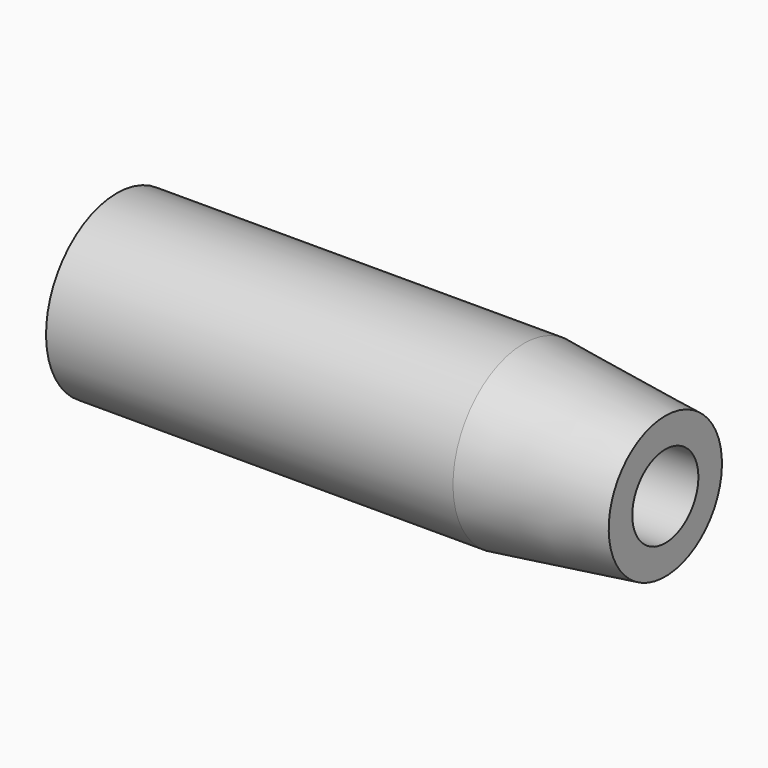
from build123d import *

# Parameters (mm, degrees)
F2_R     = 7
F3_DEPTH = 30
F5_D     = 14
F5_DEPTH = 30
F5_TIP   = 4.2060243332


with BuildPart() as f1:
    # F0 (on Front) → F1 (revolve)
    with BuildSketch(Plane.XZ):
        Polygon((-42.1976023009, 15), (-42.1976023009, 0), (-20.7868143916, 0), (26.8023976991, 0), (26.8023976991, 15), align=None)
        Polygon((26.8023976991, 15), (26.8023976991, 0), (50.8023976991, 0), (50.8023976991, 12), align=None)
    revolve(axis=Axis((4.7784452844, 0, 0), (1, 0, 0)))

    # F2 (on face) → F3 (join)
    with BuildSketch(Plane.YZ.offset(50.8023976991)):
        Circle(F2_R)
    extrude(amount=-F3_DEPTH)

    # F5
    with Locations(Plane.YZ.offset(50.8023976991)):
        with Locations((0, 0)):
            Hole(F5_D / 2, depth=F5_DEPTH)
            with Locations((0, 0, -(F5_DEPTH + F5_TIP / 2))):  # 118° drill point
                Cone(0, F5_D / 2, F5_TIP, mode=Mode.SUBTRACT)


solid = f1.part
